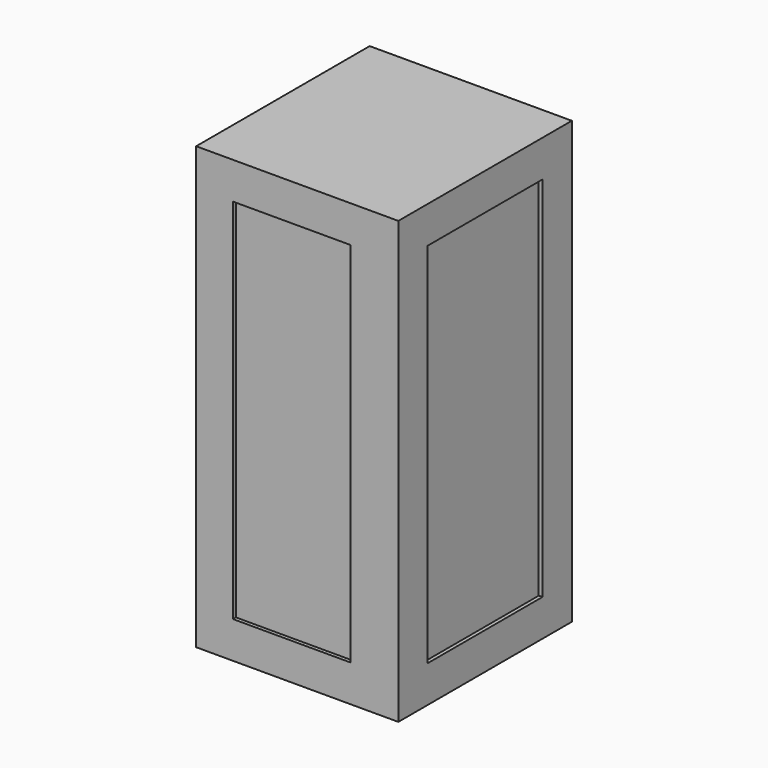
from build123d import *

# Parameters (mm, degrees)
F0_W     = 330.2
F0_H     = 762
F0_W_2   = 203.2
F0_H_2   = 635
F1_DEPTH = 374.65
F2_DEPTH = 6.35
F3_W     = 374.65
F3_H     = 762
F3_W_2   = 247.65
F3_H_2   = 635
F4_DEPTH = 19.05
F5_DEPTH = 12.7


# Not quite as in the source:
# - a feature names something its author has since deleted; it is built from what else it names


with BuildPart() as f1:
    # F0 (on Front) → F1 (new body)
    with BuildSketch(Plane.XZ):
        with Locations((48.0267770052, 381)):
            Rectangle(F0_W, F0_H)
        with Locations((48.0267770052, 381)):
            Rectangle(F0_W_2, F0_H_2, mode=Mode.SUBTRACT)
        with Locations((48.0267770052, 381)):
            Rectangle(F0_W_2, F0_H_2)
    extrude(amount=-F1_DEPTH)

    # F0 (on Front) → F2 (cut)
    with BuildSketch(Plane.XZ):
        with Locations((48.0267770052, 381)):
            Rectangle(F0_W_2, F0_H_2)
    extrude(amount=-F2_DEPTH, mode=Mode.SUBTRACT)

    # F3 (on face) → F4 (join)
    with BuildSketch(Plane.YZ.offset(213.1267770052)):
        with Locations((187.325, 381)):
            Rectangle(F3_W, F3_H)
        with Locations((187.325, 381)):
            Rectangle(F3_W_2, F3_H_2, mode=Mode.SUBTRACT)
    extrude(amount=F4_DEPTH)

    # F5 (add): a face of the model
    f5_faces = [f1.faces().sort_by_distance(p)[0] for p in [
        (213.1267770052, 187.325, 381),
    ]]
    extrude(f5_faces, amount=F5_DEPTH)


solid = f1.part
